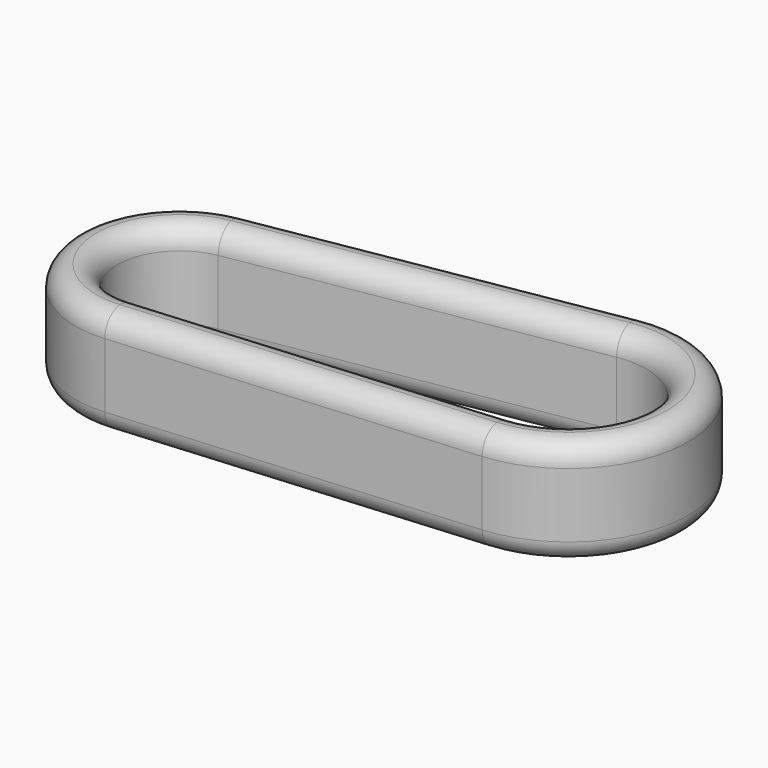
from build123d import *

# Parameters (mm, degrees)
F1_DEPTH = 25.4
F2_R     = 4.99999
F3_R     = 4.99999


# Not quite as in the source:
# - a fillet or chamfer is up to 0.001 mm smaller than in the source, because OpenCascade refuses the exact size


with BuildPart() as f1:
    # F0 (on Top) → F1 (new body)
    with BuildSketch(Plane.XY):
        with BuildLine():
            Line((33.5641757438, 33.0211686649), (-50.0175157615, 18.7475354366))
            ThreePointArc((-50.0175157615, 18.7475354366), (-70.4930751684, -8.8439952597), (-43.8361644944, -30.5223303552))
            Line((-43.8361644944, -30.5223303552), (40.6811656436, -23.7064175959))
            ThreePointArc((40.6811656436, -23.7064175959), (66.7727246476, 8.377243564), (33.5641757438, 33.0211686649))
        make_face()
        with BuildLine():
            Line((39.8773238571, -13.7387780367), (-44.640006281, -20.554690796))
            ThreePointArc((-44.640006281, -20.554690796), (-60.5708580224, -7.5991631795), (-48.3341399261, 8.8902413963))
            Line((-48.3341399261, 8.8902413963), (35.2475515791, 23.1638746246))
            ThreePointArc((35.2475515791, 23.1638746246), (56.8505075016, 7.1324114838), (39.8773238571, -13.7387780367))
        make_face(mode=Mode.SUBTRACT)
    extrude(amount=F1_DEPTH)

    # F2 (radius 5 in the source; OpenCascade refuses exactly that, so slightly less here)
    f2_edges = [f1.edges().sort_by_distance(p)[0] for p in [
        (-2.381341, -17.146734, 25.4),
        (-1.577499, -27.114374, 25.4),
    ]]
    fillet(f2_edges, radius=F2_R)

    # F3 (radius 5 in the source; OpenCascade refuses exactly that, so slightly less here)
    f3_edges = [f1.edges().sort_by_distance(p)[0] for p in [
        (-1.577499, -27.114374, 0),
        (66.772725, 8.377244, 0),
        (-8.22667, 25.884352, 0),
        (-70.493075, -8.843995, 0),
        (56.850508, 7.132411, 0),
        (-2.381341, -17.146734, 0),
        (-60.570858, -7.599163, 0),
        (-6.543294, 16.027058, 0),
    ]]
    fillet(f3_edges, radius=F3_R)


solid = f1.part
